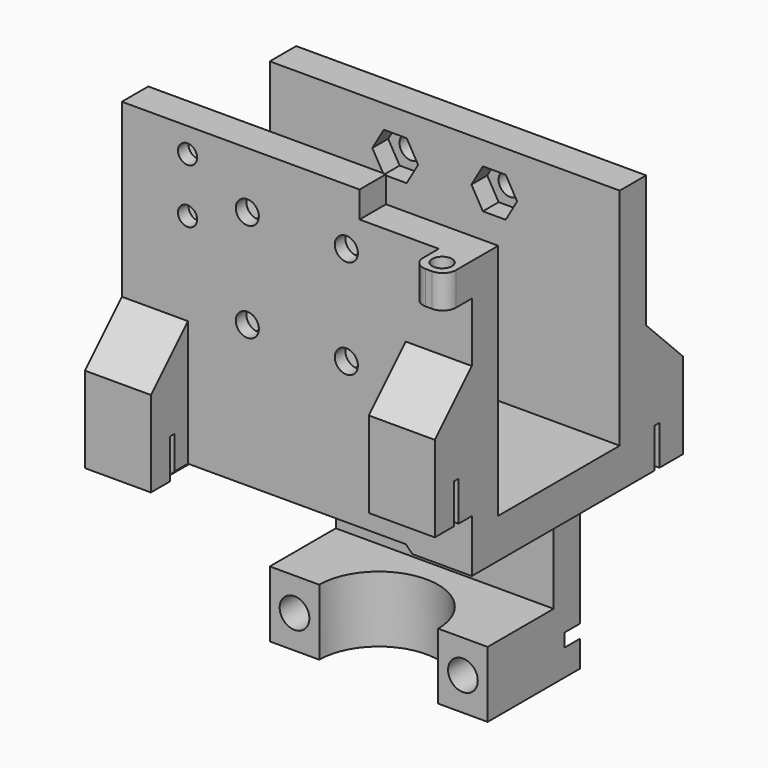
from build123d import *

# Parameters (mm, degrees)
F0_W      = 53
F0_H      = 33
F0_R      = 1.75
F1_DEPTH  = 5
F2_W      = 53
F2_H      = 5
F3_DEPTH  = 40
F4_DEPTH  = 34
F5_R      = 1.75
F6_DEPTH  = 5
F7_W      = 10
F7_H      = 20
F8_DEPTH  = 7
F9_W      = 10
F9_H      = 20
F10_DEPTH = 7
F12_DEPTH = 6
F16_DEPTH = 6
F17_DEPTH = 6
F18_DEPTH = 6
F19_R     = 1.45
F20_DEPTH = 5
F21_SIZE  = 6.99999
F22_DEPTH = 33
F23_DEPTH = 33
F24_W     = 17
F24_H     = 4
F25_DEPTH = 5
F26_W     = 5
F26_H     = 5
F27_DEPTH = 5
F28_R     = 2
F30_DEPTH = 3
F31_R     = 1.5
F32_DEPTH = 5
F33_W     = 33
F33_H     = 5
F34_DEPTH = 30
F35_W     = 33
F35_H     = 10
F36_DEPTH = 12.5
F38_DEPTH = 10
F39_R     = 2.25
F40_DEPTH = 17.5
F41_R     = 2.25
F42_DEPTH = 3
F43_R     = 1.75
F44_DEPTH = 5
F46_DEPTH = 3
F47_R     = 1.75
F48_DEPTH = 5
F49_SIZE  = 0.99999
F51_DEPTH = 3


# Not quite as in the source:
# - a fillet or chamfer is up to 0.001 mm smaller than in the source, because OpenCascade refuses the exact size
# - a feature names something its author has since deleted; it is built from what else it names


with BuildPart() as f1:
    # F0 (on Top) → F1 (new body)
    with BuildSketch(Plane.XY):
        with Locations((0, -0.5)):
            Rectangle(F0_W, F0_H)
        with Locations((-8, -7.5)):
            Circle(F0_R, mode=Mode.SUBTRACT)
        with Locations((8, -7.5)):
            Circle(F0_R, mode=Mode.SUBTRACT)
        with Locations((-8, 7.5)):
            Circle(F0_R, mode=Mode.SUBTRACT)
        with Locations((8, 7.5)):
            Circle(F0_R, mode=Mode.SUBTRACT)
    extrude(amount=F1_DEPTH)

    # F2 (on face) → F3 (join)
    with BuildSketch(Plane.XY.offset(5)):
        with Locations((0, -14.5)):
            Rectangle(F2_W, F2_H)
    extrude(amount=F3_DEPTH)

    # F2 (on face) → F4 (join)
    with BuildSketch(Plane.XY.offset(5)):
        with Locations((0, 13.5)):
            Rectangle(F2_W, F2_H)
    extrude(amount=F4_DEPTH)

    # F5 (on face) → F6 (cut)
    with BuildSketch(Plane.XZ.offset(17)):
        with Locations((-7.5, 36.43947)):
            Circle(F5_R)
        with Locations((7.5, 36.43947)):
            Circle(F5_R)
        with Locations((7.5, 21.43947)):
            Circle(F5_R)
        with Locations((-7.5, 21.43947)):
            Circle(F5_R)
    extrude(amount=-F6_DEPTH, mode=Mode.SUBTRACT)

    # F7 (on face) → F8 (join)
    with BuildSketch(Plane.XZ.offset(17)):
        with Locations((21.5, 17)):
            Rectangle(F7_W, F7_H)
        with Locations((-21.5, 9)):
            Rectangle(F7_W, F7_H)
    extrude(amount=F8_DEPTH)

    # F9 (on face) → F10 (join)
    with BuildSketch(Plane(origin=(0, 16, 0), x_dir=(-1, 0, 0), z_dir=(0, 1, 0))):
        with Locations((21.5, 17)):
            Rectangle(F9_W, F9_H)
        with Locations((-21.5, 9)):
            Rectangle(F9_W, F9_H)
    extrude(amount=F10_DEPTH)

    # F11 (on face) → F12 (cut)
    with BuildSketch(Plane(origin=(0, 0, 7), x_dir=(1, 0, 0), z_dir=(0, 0, -1))):
        Polygon((26.5, 19.5), (26.5, 20.4), (16.5, 20.4), (16.5, 19.6), (16.5, 18.6), (17.5, 18.6), (17.5, 19.5), (18.5, 19.5), (18.5, 18.6), (19.5, 18.6), (19.5, 19.5), (20.5, 19.5), (20.5, 18.6), (21.5, 18.6), (21.5, 19.5), (22.5, 19.5), (22.5, 18.6), (23.5, 18.6), (23.5, 19.5), (24.5, 19.5), (24.5, 18.6), (25.5, 18.6), (25.5, 19.5), align=None)
    extrude(amount=-F12_DEPTH, mode=Mode.SUBTRACT)

    # F15 (on face) → F16 (cut)
    with BuildSketch(Plane(origin=(0, 0, -1), x_dir=(1, 0, 0), z_dir=(0, 0, -1))):
        Polygon((-16.5, 19.5), (-16.5, 20.4), (-26.5, 20.4), (-26.5, 19.6), (-26.5, 18.6), (-25.5, 18.6), (-25.5, 19.5), (-24.5, 19.5), (-24.5, 18.6), (-23.5, 18.6), (-23.5, 19.5), (-22.5, 19.5), (-22.5, 18.6), (-21.5, 18.6), (-21.5, 19.5), (-20.5, 19.5), (-20.5, 18.6), (-19.5, 18.6), (-19.5, 19.5), (-18.5, 19.5), (-18.5, 18.6), (-17.5, 18.6), (-17.5, 19.5), align=None)
    extrude(amount=-F16_DEPTH, mode=Mode.SUBTRACT)

    # F13 (on face) → F17 (cut)
    with BuildSketch(Plane(origin=(0, 0, -1), x_dir=(1, 0, 0), z_dir=(0, 0, -1))):
        Polygon((26.5, -18.5), (26.5, -17.6), (16.5, -17.6), (16.5, -18.4), (16.5, -19.4), (17.5, -19.4), (17.5, -18.5), (18.5, -18.5), (18.5, -19.4), (19.5, -19.4), (19.5, -18.5), (20.5, -18.5), (20.5, -19.4), (21.5, -19.4), (21.5, -18.5), (22.5, -18.5), (22.5, -19.4), (23.5, -19.4), (23.5, -18.5), (24.5, -18.5), (24.5, -19.4), (25.5, -19.4), (25.5, -18.5), align=None)
    extrude(amount=-F17_DEPTH, mode=Mode.SUBTRACT)

    # F14 (on face) → F18 (cut)
    with BuildSketch(Plane(origin=(0, 0, 7), x_dir=(1, 0, 0), z_dir=(0, 0, -1))):
        Polygon((-16.5, -18.5), (-16.5, -17.6), (-26.5, -17.6), (-26.5, -18.4), (-26.5, -19.4), (-25.5, -19.4), (-25.5, -18.5), (-24.5, -18.5), (-24.5, -19.4), (-23.5, -19.4), (-23.5, -18.5), (-22.5, -18.5), (-22.5, -19.4), (-21.5, -19.4), (-21.5, -18.5), (-20.5, -18.5), (-20.5, -19.4), (-19.5, -19.4), (-19.5, -18.5), (-18.5, -18.5), (-18.5, -19.4), (-17.5, -19.4), (-17.5, -18.5), align=None)
    extrude(amount=-F18_DEPTH, mode=Mode.SUBTRACT)

    # F19 (on face) → F20 (cut)
    with BuildSketch(Plane.XZ.offset(17)):
        with Locations((-16.55, 33)):
            Circle(F19_R)
        with Locations((-16.55, 41.25)):
            Circle(F19_R)
    extrude(amount=-F20_DEPTH, mode=Mode.SUBTRACT)

    # F21 (size 7 in the source; OpenCascade refuses exactly that, so slightly less here)
    f21_edges = [f1.edges().sort_by_distance(p)[0] for p in [
        (21.5, 23, 19),
        (-21.5, 23, 27),
        (21.5, -24, 27),
        (-21.5, -24, 19),
    ]]
    chamfer(f21_edges, length=F21_SIZE)

    # F22 (add): a face of the model
    f22_faces = [f1.faces().sort_by_distance(p)[0] for p in [
        (-21.5, -17, -0.5),
    ]]
    extrude(f22_faces, amount=F22_DEPTH)

    # F23 (add): a face of the model
    f23_faces = [f1.faces().sort_by_distance(p)[0] for p in [
        (21.5, 16, -0.5),
    ]]
    extrude(f23_faces, amount=F23_DEPTH)

    # F24 (on face) → F25 (cut)
    with BuildSketch(Plane.XZ.offset(17)):
        with Locations((18, 43)):
            Rectangle(F24_W, F24_H)
    extrude(amount=-F25_DEPTH, mode=Mode.SUBTRACT)

    # F26 (on face) → F27 (join)
    with BuildSketch(Plane.XZ.offset(17)):
        with Locations((24, 38.5)):
            Rectangle(F26_W, F26_H)
    extrude(amount=F27_DEPTH)

    # F28
    f28_edges = [f1.edges().sort_by_distance(p)[0] for p in [
        (26.5, -22, 38.5),
        (21.5, -22, 38.5),
    ]]
    fillet(f28_edges, radius=F28_R)

    # F29 (on face) → F30 (cut)
    with BuildSketch(Plane(origin=(0, -12, 0), x_dir=(-1, 0, 0), z_dir=(0, 1, 0))):
        Polygon((-5.7679491924, 33.43947), (-4.0358983849, 36.43947), (-5.7679491924, 39.43947), (-9.2320508076, 39.43947), (-10.9641016151, 36.43947), (-9.2320508076, 33.43947), align=None)
        Polygon((10.9641016151, 36.43947), (9.2320508076, 39.43947), (5.7679491924, 39.43947), (4.0358983849, 36.43947), (5.7679491924, 33.43947), (9.2320508076, 33.43947), align=None)
        Polygon((5.7679491924, 18.43947), (9.2320508076, 18.43947), (10.9641016151, 21.43947), (9.2320508076, 24.43947), (5.7679491924, 24.43947), (4.0358983849, 21.43947), align=None)
        Polygon((-9.2320508076, 18.43947), (-5.7679491924, 18.43947), (-4.0358983849, 21.43947), (-5.7679491924, 24.43947), (-9.2320508076, 24.43947), (-10.9641016151, 21.43947), align=None)
        Polygon((13.0859364183, 41.2662327449), (14.8039102397, 38.2581493104), (18.2679738214, 38.2419165655), (20.0140635817, 41.2337672551), (18.2960897603, 44.2418506896), (14.8320261786, 44.2580834345), align=None)
        Polygon((14.8039102397, 35.9918506896), (13.0859364183, 32.9837672551), (14.8320261786, 29.9919165655), (18.2960897603, 30.0081493104), (20.0140635817, 33.0162327449), (18.2679738214, 36.0080834345), align=None)
    extrude(amount=-F30_DEPTH, mode=Mode.SUBTRACT)

    # F31 (on face) → F32 (cut)
    with BuildSketch(Plane(origin=(0, 0, 36), x_dir=(1, 0, 0), z_dir=(0, 0, -1))):
        with Locations((24, 19.5)):
            Circle(F31_R)
    extrude(amount=-F32_DEPTH, mode=Mode.SUBTRACT)

    # F33 (on face) → F34 (join)
    with BuildSketch(Plane(origin=(0, 0, 0), x_dir=(1, 0, 0), z_dir=(0, 0, -1))):
        with Locations((0, -13.5)):
            Rectangle(F33_W, F33_H)
    extrude(amount=F34_DEPTH)

    # F35 (on face) → F36 (join)
    with BuildSketch(Plane.XZ.offset(-11)):
        with Locations((0, -25)):
            Rectangle(F35_W, F35_H)
    extrude(amount=F36_DEPTH)

    # F37 (on face) → F38 (cut)
    with BuildSketch(Plane(origin=(0, 0, -30), x_dir=(1, 0, 0), z_dir=(0, 0, -1))):
        with BuildLine():
            ThreePointArc((-6.7779890627, 7.4210526316), (-8.4262061915, 4.6621273247), (-9, 1.5))
            Line((-9, 1.5), (9, 1.5))
            ThreePointArc((9, 1.5), (3.1621273247, 9.9262061915), (-6.7779890627, 7.4210526316))
        make_face()
        with BuildLine():
            Line((9, 1.5), (-9, 1.5))
            ThreePointArc((-9, 1.5), (-3.3702186642, -6.8451558497), (6.4759169235, -4.75))
            ThreePointArc((6.4759169235, -4.75), (8.3451558497, -1.8702186642), (9, 1.5))
        make_face()
    extrude(amount=-F38_DEPTH, mode=Mode.SUBTRACT)

    # F39 (on face) → F40 (cut)
    with BuildSketch(Plane.XZ.offset(1.5)):
        with Locations((-12.75, -25)):
            Circle(F39_R)
        with Locations((12.75, -25)):
            Circle(F39_R)
    extrude(amount=-F40_DEPTH, mode=Mode.SUBTRACT)

    # F41 (on face) → F42 (cut)
    with BuildSketch(Plane(origin=(0, 16, 0), x_dir=(-1, 0, 0), z_dir=(0, 1, 0))):
        Polygon((-8.4198729811, -25), (-10.5849364905, -21.25), (-14.9150635095, -21.25), (-16.5, -23.9951905284), (-16.5, -26.0048094716), (-14.9150635095, -28.75), (-10.5849364905, -28.75), align=None)
        with Locations((-12.75, -25)):
            Circle(F41_R, mode=Mode.SUBTRACT)
        Polygon((14.9150635095, -28.75), (16.5, -26.0048094716), (16.5, -23.9951905284), (14.9150635095, -21.25), (10.5849364905, -21.25), (8.4198729811, -25), (10.5849364905, -28.75), align=None)
        with Locations((12.75, -25)):
            Circle(F41_R, mode=Mode.SUBTRACT)
    extrude(amount=-F42_DEPTH, mode=Mode.SUBTRACT)

    # F43 (on face) → F44 (cut)
    with BuildSketch(Plane(origin=(0, 16, 0), x_dir=(-1, 0, 0), z_dir=(0, 1, 0))):
        with Locations((-7.5, -7.5)):
            Circle(F43_R)
        with Locations((7.5, -7.5)):
            Circle(F43_R)
    extrude(amount=-F44_DEPTH, mode=Mode.SUBTRACT)

    # F45 (on face) → F46 (cut)
    with BuildSketch(Plane.XZ.offset(-11)):
        Polygon((-10.9641016151, -7.5), (-9.2320508076, -10.5), (-5.7679491924, -10.5), (-4.0358983849, -7.5), (-5.7679491924, -4.5), (-9.2320508076, -4.5), align=None)
        Polygon((5.7679491924, -10.5), (9.2320508076, -10.5), (10.9641016151, -7.5), (9.2320508076, -4.5), (5.7679491924, -4.5), (4.0358983849, -7.5), align=None)
    extrude(amount=-F46_DEPTH, mode=Mode.SUBTRACT)

    # F47 (on face) → F48 (cut)
    with BuildSketch(Plane(origin=(0, 16, 0), x_dir=(-1, 0, 0), z_dir=(0, 1, 0))):
        with Locations((7.5, 32.5)):
            Circle(F47_R)
        with Locations((-7.5, 32.5)):
            Circle(F47_R)
    extrude(amount=-F48_DEPTH, mode=Mode.SUBTRACT)

    # F49 (size 1 in the source; OpenCascade refuses exactly that, so slightly less here)
    f49_edges = [f1.edges().sort_by_distance(p)[0] for p in [
        (16.5, -3, -1),
        (-16.5, -4.25, -1),
    ]]
    chamfer(f49_edges, length=F49_SIZE)

    # F50 (on face) → F51 (cut)
    with BuildSketch(Plane.XZ.offset(-11)):
        Polygon((9.2320508076, 35.5), (5.7679491924, 35.5), (4.0358983849, 32.5), (5.7679491924, 29.5), (9.2320508076, 29.5), (10.9641016151, 32.5), align=None)
        Polygon((-9.2320508076, 35.5), (-10.9641016151, 32.5), (-9.2320508076, 29.5), (-5.7679491924, 29.5), (-4.0358983849, 32.5), (-5.7679491924, 35.5), align=None)
    extrude(amount=-F51_DEPTH, mode=Mode.SUBTRACT)


solid = f1.part
